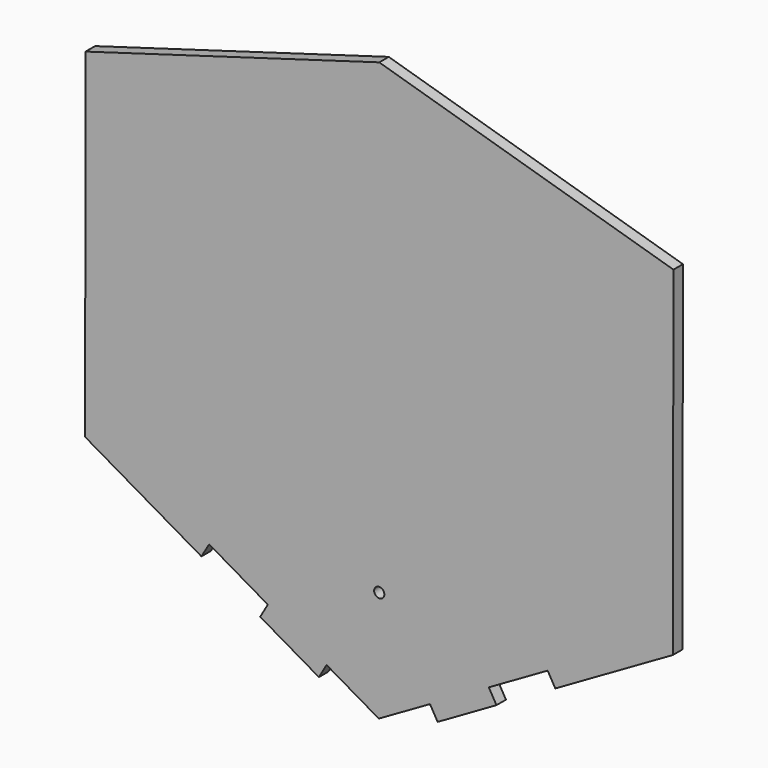
from build123d import *

# Parameters (mm, degrees)
F1_DEPTH = 3.5
F2_R     = 1.5
F3_DEPTH = 25


# Not quite as in the source:
# - a feature names something its author has since deleted; it is built from what else it names


with BuildPart() as f1:
    # F0 (on Front) → F1 (new body)
    with BuildSketch(Plane.XZ):
        Polygon((0, 75.4606574774), (-86.5353767039, 50.1161508768), (-86.6695481512, -49.8837591133), (-0.1341714472, -99.9999099901), (86.5353767039, -50.1161508768), (86.6695481512, 49.8837591133), align=None)
    extrude(amount=F1_DEPTH)

    # F2 (on face) → F3 (cut)
    with BuildSketch(Plane.XZ.offset(3.5)):
        Polygon((0.1341714472, 99.9999099901), (-17.199738183, 90.0231581674), (-14.9549690229, 86.1230285006), (0.1271996943, 94.8037622444), (-2.1236443549, 96.1073174408), align=None)
        Polygon((17.4386577754, 89.9781792171), (0.1341714472, 99.9999099901), (2.3789406073, 96.0997803233), (0.1271996943, 94.8037622444), (15.1834309859, 86.0840872654), align=None)
        Polygon((2.3789406073, 96.0997803233), (0.1341714472, 99.9999099901), (-2.1236443549, 96.1073174408), (0.1271996943, 94.8037622444), align=None)
        Polygon((-50.1288800257, -65.8258142354), (-52.3961295985, -69.7328876509), (-35.0856874223, -79.7580676974), (-32.8304606328, -75.8639757457), align=None)
        Polygon((-15.5233852921, -85.8872059211), (-17.7786120815, -89.7812978727), (-0.4715367407, -99.8045280481), (-0.3587329239, -99.6097501051), (-2.3789406073, -96.0997803233), (-0.1271996943, -94.8037622444), align=None)
        Polygon((-0.3587329239, -99.6097501051), (-0.4715367407, -99.8045280481), (-0.1341714472, -99.9999099901), align=None)
        Polygon((14.9549690229, -86.1230285006), (-0.1271996943, -94.8037622444), (1.7836900487, -95.9104360964), (-0.3587329239, -99.6097501051), (-0.1341714472, -99.9999099901), (17.199738183, -90.0231581674), align=None)
        Polygon((1.7836900487, -95.9104360964), (-0.1271996943, -94.8037622444), (-2.3789406073, -96.0997803233), (-0.3587329239, -99.6097501051), align=None)
        Polygon((34.5336478132, -80.0464063448), (51.8675574435, -70.0696545221), (49.6227882834, -66.1695248553), (32.2888786531, -76.146276678), align=None)
        with Locations((0, -62.0760797054)):
            Circle(F2_R)
    extrude(amount=-F3_DEPTH, mode=Mode.SUBTRACT)


solid = f1.part
